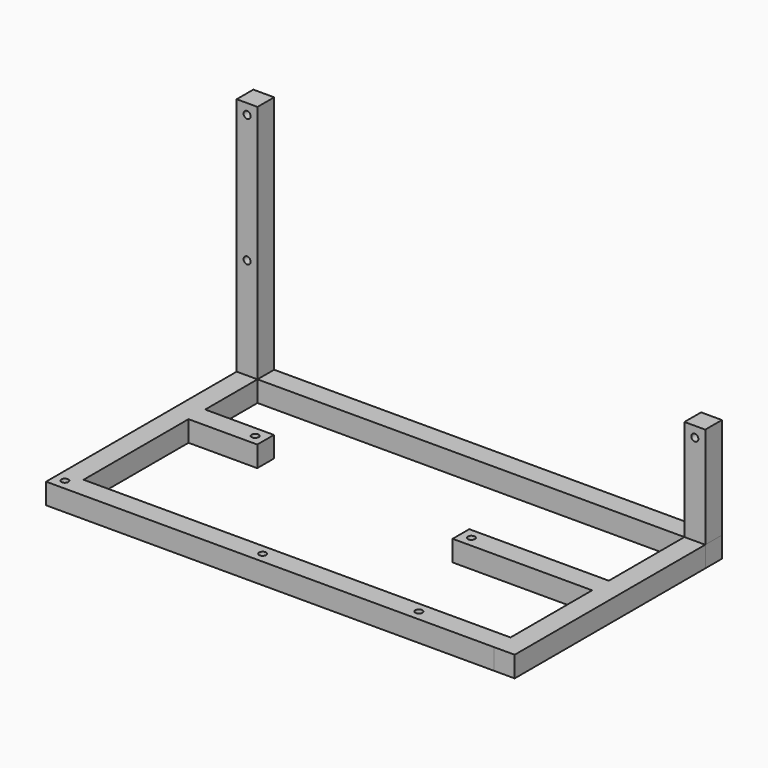
from build123d import *

# Parameters (mm, degrees)
F0_R      = 4.318
F0_W      = 260.35
F0_H      = 12.7
F0_W_2    = 41.9088844856
F0_W_3    = 12.695625494
F0_W_4    = 85.0911155144
F0_R_2    = 2.159
F1_DEPTH  = 12.7
F2_W      = 12.7
F2_H      = 12.7
F3_DEPTH  = 146.2532
F2_W_2    = 12.695625494
F4_DEPTH  = 61.7982
F6_R      = 2.159
F7_DEPTH  = 12.7
F5_R      = 2.159
F8_DEPTH  = 12.7
F6_R_2    = 4.318
F9_DEPTH  = 6.35
F5_R_2    = 4.318
F10_DEPTH = 6.35
F11_DEPTH = 6.35


# Not quite as in the source:
# - a feature names something its author has since deleted; it is built from what else it names


with BuildPart() as f1:
    # F0 (on Top) → F1 (new body)
    with BuildSketch(Plane.XY):
        Polygon((-142.8771033979, -6.35), (-142.8756433805, -151.63), (-130.175, -151.63), (-130.175, -138.93), (-130.175, -58.92), (-130.175, -46.22), (-130.175, -6.35), align=None)
        with Locations((-136.5261155144, -145.28)):
            Circle(F0_R, mode=Mode.SUBTRACT)
        with Locations((0, -145.28)):
            Rectangle(F0_W, F0_H)
        with Locations((-15.8761155144, -145.28)):
            Circle(F0_R, mode=Mode.SUBTRACT)
        with Locations((79.3738844856, -145.28)):
            Circle(F0_R, mode=Mode.SUBTRACT)
        Polygon((-142.8772310289, 6.35), (-142.8771033979, -6.35), (-130.175, -6.35), (-130.175, 6.35), align=None)
        Polygon((130.175, -138.93), (130.175, -151.63), (142.8736619349, -151.6297345897), (142.870625494, -6.35), (130.175, -6.35), (130.175, -64), (130.175, -76.7), align=None)
        Rectangle(F0_W, F0_H)
        with Locations((-109.2205577572, -52.57)):
            Rectangle(F0_W_2, F0_H)
        with Locations((-94.6161155144, -52.57)):
            Circle(F0_R, mode=Mode.SUBTRACT)
        with Locations((136.522812747, 0)):
            Rectangle(F0_W_3, F0_H)
        with Locations((87.6294422428, -70.35)):
            Rectangle(F0_W_4, F0_H)
        with Locations((51.4338844856, -70.35)):
            Circle(F0_R, mode=Mode.SUBTRACT)
        with Locations((-94.6161155144, -52.57)):
            Circle(F0_R)
        with Locations((-94.6161155144, -52.57)):
            Circle(F0_R_2, mode=Mode.SUBTRACT)
        with Locations((51.4338844856, -70.35)):
            Circle(F0_R)
        with Locations((51.4338844856, -70.35)):
            Circle(F0_R_2, mode=Mode.SUBTRACT)
        with Locations((-136.5261155144, -145.28)):
            Circle(F0_R)
        with Locations((-136.5261155144, -145.28)):
            Circle(F0_R_2, mode=Mode.SUBTRACT)
        with Locations((-15.8761155144, -145.28)):
            Circle(F0_R)
        with Locations((-15.8761155144, -145.28)):
            Circle(F0_R_2, mode=Mode.SUBTRACT)
        with Locations((79.3738844856, -145.28)):
            Circle(F0_R)
        with Locations((79.3738844856, -145.28)):
            Circle(F0_R_2, mode=Mode.SUBTRACT)
    extrude(amount=F1_DEPTH)

    # F0 (on Top) → F11 (cut)
    with BuildSketch(Plane.XY):
        with Locations((-136.5261155144, -145.28)):
            Circle(F0_R)
        with Locations((-136.5261155144, -145.28)):
            Circle(F0_R_2, mode=Mode.SUBTRACT)
        with Locations((-15.8761155144, -145.28)):
            Circle(F0_R)
        with Locations((-15.8761155144, -145.28)):
            Circle(F0_R_2, mode=Mode.SUBTRACT)
        with Locations((79.3738844856, -145.28)):
            Circle(F0_R)
        with Locations((79.3738844856, -145.28)):
            Circle(F0_R_2, mode=Mode.SUBTRACT)
        with Locations((51.4338844856, -70.35)):
            Circle(F0_R)
        with Locations((51.4338844856, -70.35)):
            Circle(F0_R_2, mode=Mode.SUBTRACT)
        with Locations((-94.6161155144, -52.57)):
            Circle(F0_R)
        with Locations((-94.6161155144, -52.57)):
            Circle(F0_R_2, mode=Mode.SUBTRACT)
    extrude(amount=F11_DEPTH, mode=Mode.SUBTRACT)


with BuildPart() as f3:
    # F2 (on face) → F3 (new body)
    with BuildSketch(Plane.XY.offset(12.7)):
        with Locations((-136.525, 0)):
            Rectangle(F2_W, F2_H)
    extrude(amount=F3_DEPTH)

    # F5 (on face) → F8 (cut, through all)
    with BuildSketch(Plane(origin=(0, 6.35, 0), x_dir=(-1, 0, 0), z_dir=(0, 1, 0))):
        with Locations((136.525, 152.6032)):
            Circle(F5_R)
        with Locations((136.525, 74.4982)):
            Circle(F5_R)
    extrude(amount=-F8_DEPTH, mode=Mode.SUBTRACT)

    # F5 (on face) → F10 (cut)
    with BuildSketch(Plane(origin=(0, 6.35, 0), x_dir=(-1, 0, 0), z_dir=(0, 1, 0))):
        with Locations((136.525, 152.6032)):
            Circle(F5_R_2)
        with Locations((136.525, 152.6032)):
            Circle(F5_R, mode=Mode.SUBTRACT)
        with Locations((136.525, 74.4982)):
            Circle(F5_R_2)
        with Locations((136.525, 74.4982)):
            Circle(F5_R, mode=Mode.SUBTRACT)
    extrude(amount=-F10_DEPTH, mode=Mode.SUBTRACT)


with BuildPart() as f4:
    # F2 (on face) → F4 (new body)
    with BuildSketch(Plane.XY.offset(12.7)):
        with Locations((136.522812747, 0)):
            Rectangle(F2_W_2, F2_H)
    extrude(amount=F4_DEPTH)

    # F6 (on face) → F7 (cut, through all)
    with BuildSketch(Plane(origin=(0, 6.35, 0), x_dir=(-1, 0, 0), z_dir=(0, 1, 0))):
        with Locations((-136.525, 68.1482)):
            Circle(F6_R)
    extrude(amount=-F7_DEPTH, mode=Mode.SUBTRACT)

    # F6 (on face) → F9 (cut)
    with BuildSketch(Plane(origin=(0, 6.35, 0), x_dir=(-1, 0, 0), z_dir=(0, 1, 0))):
        with Locations((-136.525, 68.1482)):
            Circle(F6_R_2)
        with Locations((-136.525, 68.1482)):
            Circle(F6_R, mode=Mode.SUBTRACT)
    extrude(amount=-F9_DEPTH, mode=Mode.SUBTRACT)


solid = Compound([f1.part, f3.part, f4.part])
